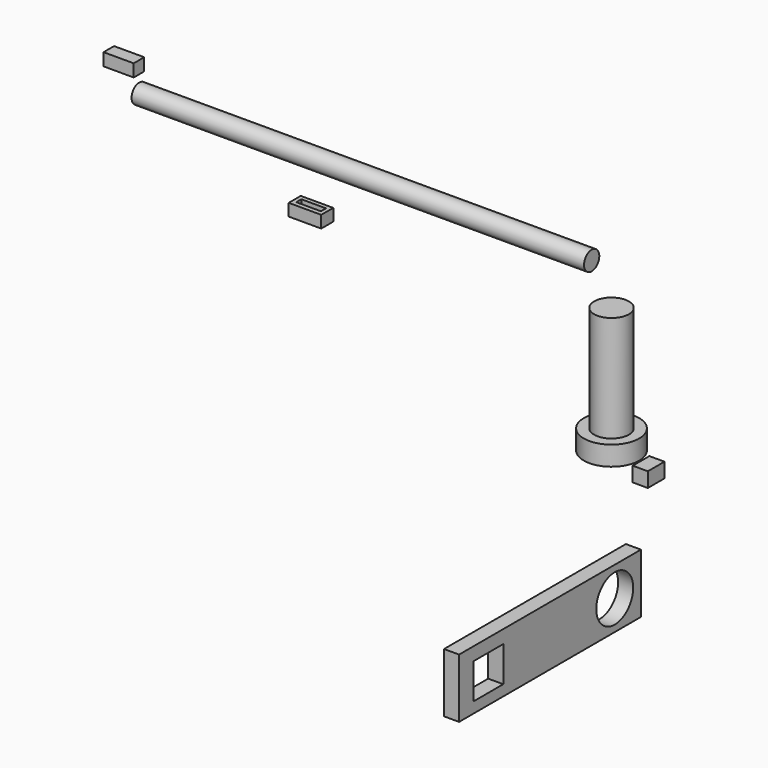
from build123d import *

# Parameters (mm, degrees)
F0_W      = 4.6600201167
F0_H      = 21.1479533464
F2_W      = 76.2
F2_H      = 1.6046876216
F4_W      = 2.5020283647
F4_H      = 18.3248373214
F6_W      = 2.2167799762
F6_H      = 2.1073091775
F7_DEPTH  = 5.08
F10_W     = 38.2821860258
F10_H     = 9.9848276004
F10_W_2   = 6.2995692715
F10_H_2   = 5.9559568763
F10_R     = 3.8874076759
F11_DEPTH = 2.54
F12_W     = 3.4997598268
F12_H     = 2.4837013334
F13_DEPTH = 2.54
F14_W     = 5.4736100137
F14_H     = 2.0410064608
F15_DEPTH = 2.54
F16_W     = 4.1583329439
F16_H     = 1.0704973829
F17_DEPTH = 13.3158767054


# Not quite as in the source:
# - a feature of the source that left no trace in its solid (it failed there, or was rolled back) is left out


with BuildPart() as f1:
    # F0 (on Front) → F1 (revolve)
    with BuildSketch(Plane.XZ):
        with Locations((-2.3300100584, 10.5739766732)):
            Rectangle(F0_W, F0_H)
    revolve(axis=Axis((0, 0, 10.5739766732), (0, 0, -1)))

    # F4 (on Front) → F5 (revolve, cut)
    with BuildSketch(Plane.XZ):
        with Locations((4.1766406503, 12.4440173386)):
            Rectangle(F4_W, F4_H)
    revolve(axis=Axis((0, 0, 21.1479533464), (0, 0, -1)), mode=Mode.SUBTRACT)


with BuildPart() as f3:
    # F2 (on Front) → F3 (revolve)
    with BuildSketch(Plane.XZ):
        with Locations((-41.4429178875, 27.8707629937)):
            Rectangle(F2_W, F2_H)
    revolve(axis=Axis((-41.4429178875, 0, 27.0684191829), (1, 0, 0)))


with BuildPart() as f7:
    # F6 (on face) → F7 (new body)
    with BuildSketch(Plane(origin=(-79.5429178875, 0, 0), x_dir=(0, -1, 0), z_dir=(-1, 0, 0))):
        with Locations((0.046658155, 30.9424130246)):
            Rectangle(F6_W, F6_H)
    extrude(amount=F7_DEPTH)


with BuildPart() as f11:
    # F10 (on Right) → F11 (new body)
    with BuildSketch(Plane.YZ):
        with Locations((-16.1193663953, -20.1010354795)):
            Rectangle(F10_W, F10_H)
        with Locations((-29.1127148084, -20.3032046556)):
            Rectangle(F10_W_2, F10_H_2, mode=Mode.SUBTRACT)
        with Locations((-2.4962052703, -20.1010350138)):
            Circle(F10_R, mode=Mode.SUBTRACT)
    extrude(amount=F11_DEPTH)


with BuildPart() as f13:
    # F12 (on Right) → F13 (new body)
    with BuildSketch(Plane.YZ):
        with Locations((6.2213118654, -5.3245727904)):
            Rectangle(F12_W, F12_H)
    extrude(amount=F13_DEPTH)


with BuildPart() as f15:
    # F14 (on Front) → F15 (new body)
    with BuildSketch(Plane.XZ):
        with Locations((-49.5937671512, 19.7016941383)):
            Rectangle(F14_W, F14_H)
    extrude(amount=F15_DEPTH)

    # F16 (on face) → F17 (cut, through all)
    with BuildSketch(Plane(origin=(0, 0, 18.681190908), x_dir=(1, 0, 0), z_dir=(0, 0, -1))):
        with Locations((-49.5957992971, 1.2363959977)):
            Rectangle(F16_W, F16_H)
    extrude(amount=-F17_DEPTH, mode=Mode.SUBTRACT)


solid = Compound([f1.part, f3.part, f7.part, f11.part, f13.part, f15.part])
